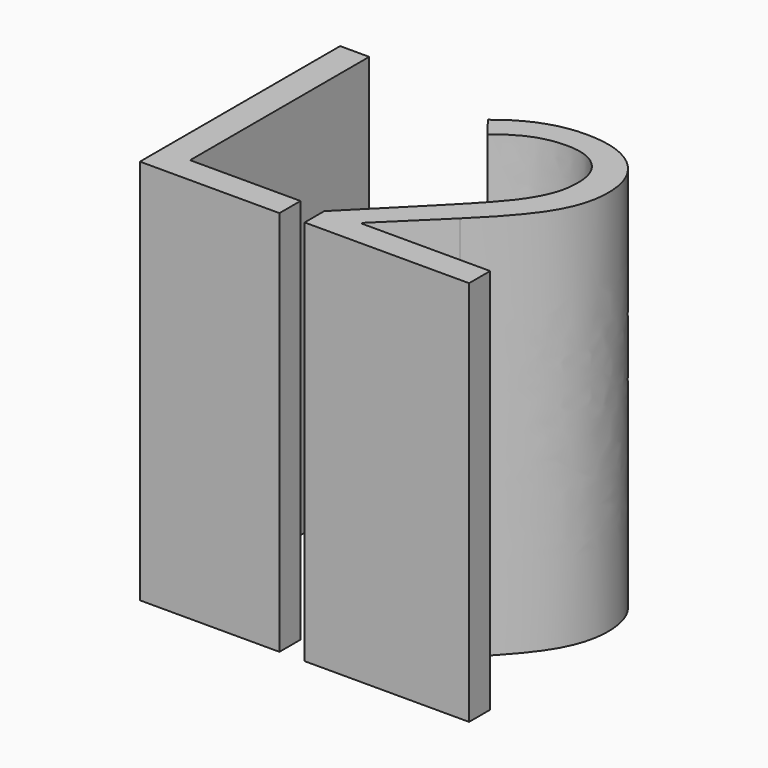
from build123d import *

# Parameters (mm, degrees)
F0_TEXT_SIZE = 9.0741528428
F1_DEPTH     = 10


# Not quite as in the source:
# - Text() gives the source's letters only with a copy of the font that has no kerning and outlines rounded to 1/6400 em; it was checked with that copy


with BuildPart() as f1:
    # F0 (on Top) → F1 (new body)
    with BuildSketch(Plane.XY):
        with Locations((-5, -3.2666950234)):
            Text('L2', F0_TEXT_SIZE, font='Open Sans', text_align=(TextAlign.LEFT, TextAlign.BOTTOM))
    extrude(amount=F1_DEPTH)


solid = f1.part
